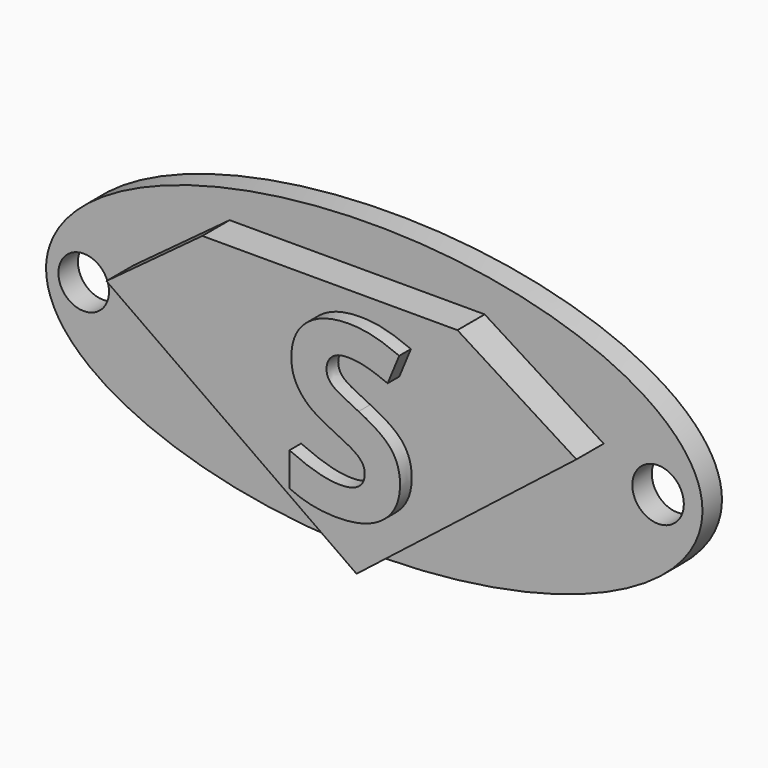
from build123d import *

# Parameters (mm, degrees)
F1_DEPTH     = 5
F3_DEPTH     = 7
F4_TEXT_SIZE = 48.7769821272
F5_DEPTH     = 3
F6_R         = 5.1916142551
F6_R_2       = 5.2846567887
F7_DEPTH     = 25


# Not quite as in the source:
# - Text() gives the source's letters only with a copy of the font that has no kerning and outlines rounded to 1/6400 em; it was checked with that copy


with BuildPart() as f1:
    # F0 (on Front) → F1 (new body)
    with BuildSketch(Plane.XZ):
        with BuildLine():
            add(Edge.make_bspline(
                [(-67.3167929053, 0), (-67.3167929053, -51.5760049336), (33.6583964527, -25.7880024668), (134.6335858107, 0), (33.6583964527, 25.7880024668), (-67.3167929053, 51.5760049336), (-67.3167929053, 0)],
                knots=[0, 0, 0, 2.0943951024, 2.0943951024, 4.1887902048, 4.1887902048, 6.2831853072, 6.2831853072, 6.2831853072], degree=2, weights=[1, 0.5, 1, 0.5, 1, 0.5, 1]))
        make_face()
    extrude(amount=F1_DEPTH)

    # F2 (on face) → F3 (join)
    with BuildSketch(Plane.XZ.offset(5)):
        Polygon((47.0647066832, 5.5621922947), (22.6571247348, 20.9651887417), (-29.6650268137, 20.9651887417), (-49.3466295302, 6.4179147594), (1.9679007799, -29.7646938183), align=None)
    extrude(amount=F3_DEPTH)

    # F4 (on face) → F5 (join)
    with BuildSketch(Plane.XZ.offset(12)):
        with Locations((-11.6502182405, -18.4201252525)):
            Text('S', F4_TEXT_SIZE, font='Open Sans', font_style=FontStyle.BOLD, text_align=(TextAlign.LEFT, TextAlign.BOTTOM))
    extrude(amount=F5_DEPTH)

    # F6 (on face) → F7 (cut)
    with BuildSketch(Plane.XZ.offset(5)):
        with Locations((-59.5950335264, 0)):
            Circle(F6_R)
        with Locations((58.2189559937, 0)):
            Circle(F6_R_2)
    extrude(amount=-F7_DEPTH, mode=Mode.SUBTRACT)


solid = f1.part
